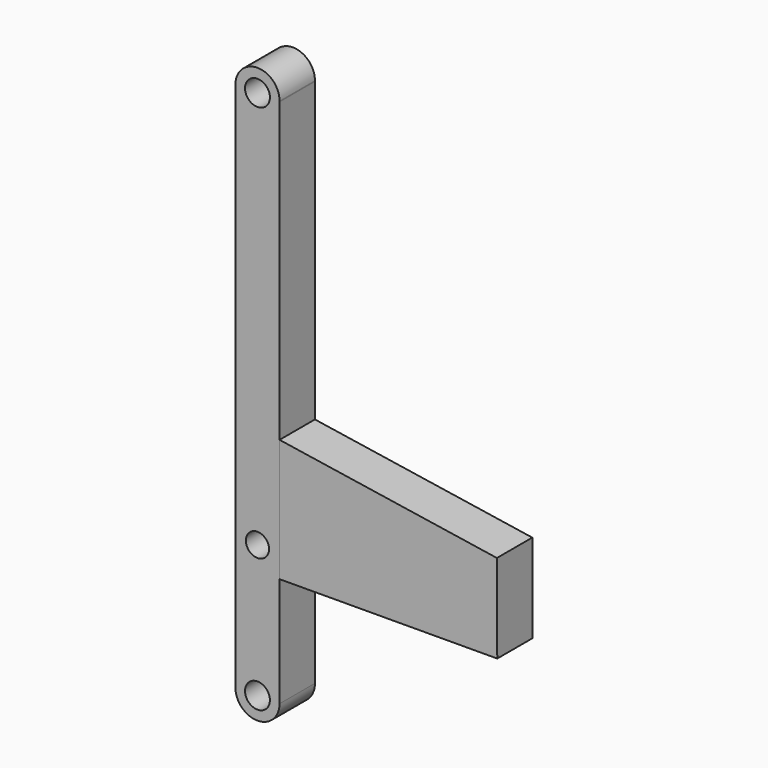
from build123d import *

# Parameters (mm, degrees)
F0_R     = 7.1501
F0_R_2   = 6.646798642
F0_R_3   = 7.1470953858
F1_DEPTH = 25.4


# Not quite as in the source:
# - a feature names something its author has since deleted; it is built from what else it names


with BuildPart() as f1:
    # F0 (on Front) → F1 (new body)
    with BuildSketch(Plane.XZ):
        with BuildLine():
            ThreePointArc((12.692106418, -0.4476993117), (12.6980264512, -0.223884447), (12.7, 0))
            ThreePointArc((12.7, 0), (0, 12.7), (-12.7, 0))
            ThreePointArc((-12.7, 0), (-0.223884447, -12.6980264512), (12.692106418, -0.4476993117))
        make_face()
        Circle(F0_R, mode=Mode.SUBTRACT)
        with BuildLine():
            ThreePointArc((12.692106418, -0.4476993117), (-0.223884447, -12.6980264512), (-12.7, 0))
            Line((-12.7, 0), (-12.7, -304.8))
            ThreePointArc((-12.7, -304.8), (-0.0001646916, -292.1000000011), (12.6999999957, -304.7996706168))
            Line((12.6999999957, -304.7996706168), (12.6983662356, -241.8069263698))
            Line((12.6983662356, -241.8069263698), (12.6980129786, -241.8069278017))
            Line((12.6980129786, -241.8069278017), (12.6980129786, -228.1864268658))
            Line((12.6980129786, -228.1864268658), (12.6965389522, -171.3525252163))
            Line((12.6965389522, -171.3525252163), (12.692106418, -0.4476993117))
        make_face()
        with Locations((0, -228.6)):
            Circle(F0_R_2, mode=Mode.SUBTRACT)
        with BuildLine():
            ThreePointArc((12.6999999957, -304.7996706168), (-0.0001646916, -292.1000000011), (-12.7, -304.8))
            ThreePointArc((-12.7, -304.8), (0, -317.5), (12.7, -304.8))
            ThreePointArc((12.7, -304.8), (12.6999999989, -304.7998353084), (12.6999999957, -304.7996706168))
        make_face()
        with Locations((0, -304.8)):
            Circle(F0_R_3, mode=Mode.SUBTRACT)
    extrude(amount=F1_DEPTH)


with BuildPart() as f1b:
    # F0 (on Front) → F1, piece 2 (new body)
    with BuildSketch(Plane.XZ):
        Polygon((137.5501584362, -190.5), (12.7, -171.3530560005), (12.7, -241.8069197473), (137.7560782405, -241.3), align=None)
    extrude(amount=F1_DEPTH)


solid = Compound([f1.part, f1b.part])
